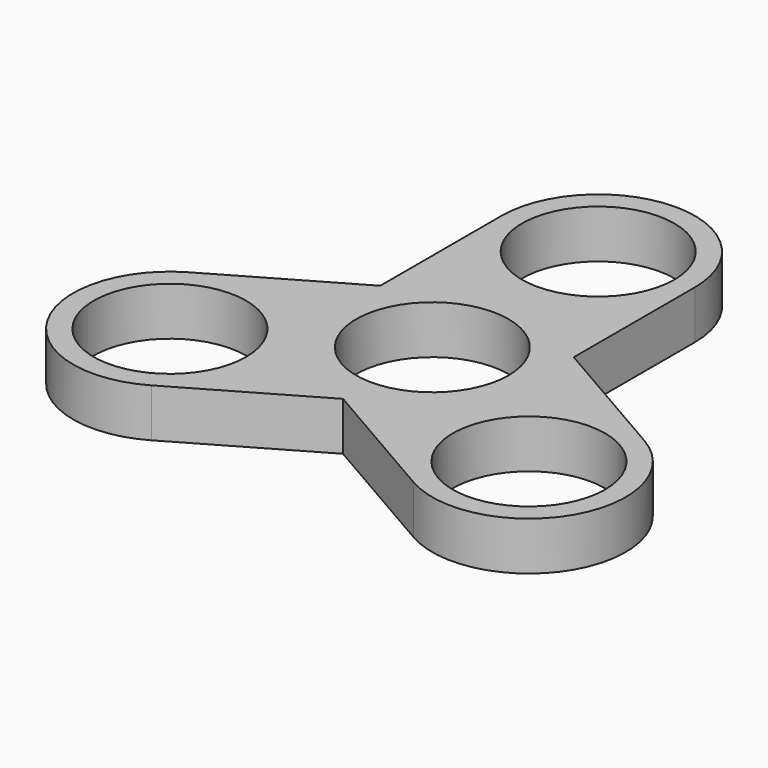
from build123d import *

# Parameters (mm, degrees)
F1_DEPTH        = 177.8
F1_COPIES_COUNT = 3


# Not quite as in the source:
# - a feature of the source that left no trace in its solid (it failed there, or was rolled back) is left out
# - a pattern or mirror of a feature is missing from the dataset's text; its kind, count and spacing are read off the source's solid


with BuildPart() as f1:
    # F0 (on Top) → F1 (new body)
    with BuildSketch(Plane.XY):
        with BuildLine():
            ThreePointArc((75.565, 0), (355.6, 280.035), (635.635, 0))
            Line((635.635, 0), (711.2, 0))
            ThreePointArc((711.2, 0), (355.6, 355.6), (0, 0))
            Line((0, 0), (75.565, 0))
        make_face()
        with BuildLine():
            Line((711.2, 0), (635.635, 0))
            ThreePointArc((635.635, 0), (355.6, -280.035), (75.565, 0))
            Line((75.565, 0), (0, 0))
            ThreePointArc((0, 0), (355.6, -355.6), (711.2, 0))
        make_face()
        with BuildLine():
            Line((711.2, -762), (711.2, 0))
            ThreePointArc((711.2, 0), (355.6, -355.6), (0, 0))
            Line((0, 0), (0, -762))
            ThreePointArc((0, -762), (355.6, -406.4), (711.2, -762))
        make_face()
        with BuildLine():
            ThreePointArc((0, -762), (355.6, -1117.6), (711.2, -762))
            Line((711.2, -762), (635.635, -762))
            ThreePointArc((635.635, -762), (355.6, -1042.035), (75.565, -762))
            Line((75.565, -762), (0, -762))
        make_face()
        with BuildLine():
            Line((635.635, -762), (711.2, -762))
            ThreePointArc((711.2, -762), (355.6, -406.4), (0, -762))
            Line((0, -762), (75.565, -762))
            ThreePointArc((75.565, -762), (355.6, -481.965), (635.635, -762))
        make_face()
    extrude(amount=F1_DEPTH)

    # F1_copies: F1 ×3 about axis
    f1_copies_axis = Axis((355.6, -762, 0), (0, 0, 1))


with BuildPart() as f1_1:
    add(f1.part)
    for i in range(1, F1_COPIES_COUNT):
        add(f1.part.rotate(f1_copies_axis, i * 360 / F1_COPIES_COUNT))


solid = f1_1.part
